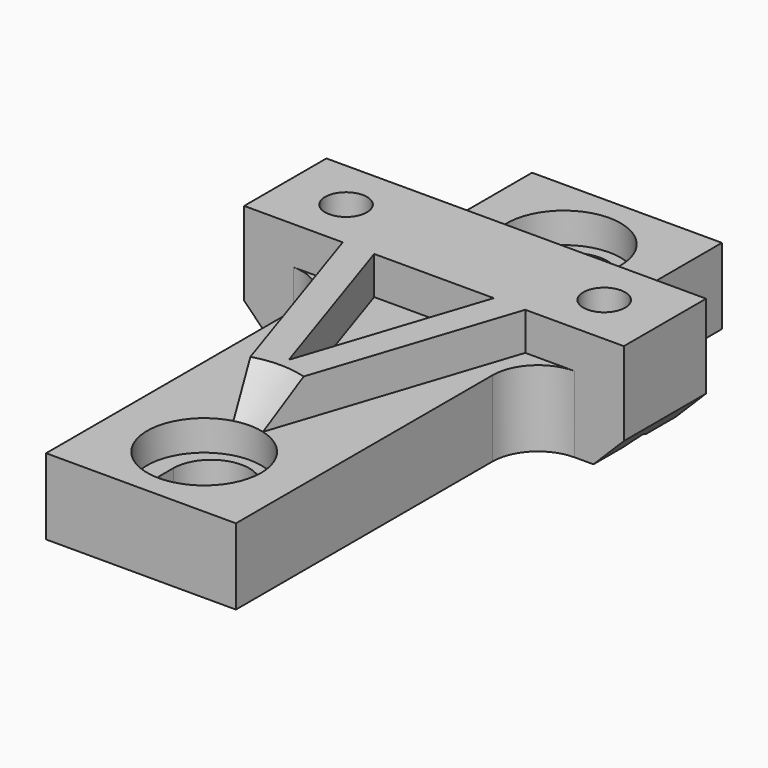
from build123d import *

# Parameters (mm, degrees)
F0_W          = 15.875
F0_H          = 50.8
F1_DEPTH      = 6.35
F2_W          = 31.75
F2_H          = 8.6
F2_R          = 1.75
F3_DEPTH      = 3.175
F3_DEPTH_BACK = 6.35
F4_R          = 4.7625
F5_DEPTH      = 2.54
F6_SIZE       = 2.54
F8_DEPTH      = 5.08
F9_R          = 3.81
F11_DEPTH     = 3.175
F12_SIZE      = 3.17499


# Not quite as in the source:
# - a fillet or chamfer is up to 0.001 mm smaller than in the source, because OpenCascade refuses the exact size


with BuildPart() as f1:
    # F0 (on Top) → F1 (new body)
    with BuildSketch(Plane.XY):
        Rectangle(F0_W, F0_H)
        with BuildLine():
            ThreePointArc((-3.175, -18.058110271), (0.0514516208, -14.8835271912), (3.1733324288, -18.161))
            Line((3.1733324288, -18.161), (3.1733324288, -19.431))
            ThreePointArc((3.1733324288, -19.431), (-0.053119192, -22.6055830798), (-3.175, -19.328110271))
            Line((-3.175, -19.328110271), (-3.175, -18.058110271))
        make_face(mode=Mode.SUBTRACT)
        with BuildLine():
            ThreePointArc((3.1733324288, 18.161), (0.0514516208, 14.8835271912), (-3.175, 18.058110271))
            Line((-3.175, 18.058110271), (-3.175, 19.328110271))
            ThreePointArc((-3.175, 19.328110271), (-0.053119192, 22.6055830798), (3.1733324288, 19.431))
            Line((3.1733324288, 19.431), (3.1733324288, 18.161))
        make_face(mode=Mode.SUBTRACT)
    extrude(amount=F1_DEPTH)

    # F2 (on face) → F3 (join, two sides)
    with BuildSketch(Plane.XY.offset(6.35)) as f3_sk:
        with Locations((0, 9.525)):
            Rectangle(F2_W, F2_H)
        with Locations((-10.795, 9.525)):
            Circle(F2_R, mode=Mode.SUBTRACT)
        with Locations((10.795, 9.525)):
            Circle(F2_R, mode=Mode.SUBTRACT)
    extrude(amount=F3_DEPTH)
    extrude(f3_sk.sketch, amount=-F3_DEPTH_BACK)

    # F4 (on face) → F5 (cut)
    with BuildSketch(Plane.XY.offset(6.35)):
        with Locations((0, -18.796)):
            Circle(F4_R)
        with Locations((0, 18.796)):
            Circle(F4_R)
    extrude(amount=-F5_DEPTH, mode=Mode.SUBTRACT)

    # F6
    f6_edges = [f1.edges().sort_by_distance(p)[0] for p in [
        (-15.875, 9.525, 0),
        (15.875, 9.525, 0),
    ]]
    chamfer(f6_edges, length=F6_SIZE)

    # F7 (on face) → F8 (cut)
    with BuildSketch(Plane(origin=(0, 0, 0), x_dir=(1, 0, 0), z_dir=(0, 0, -1))):
        Polygon((-9.1818833479, -12.319), (-7.5687666958, -9.525), (-9.1818833479, -6.731), (-12.4081166521, -6.731), (-14.0212333042, -9.525), (-12.4081166521, -12.319), align=None)
        Polygon((12.4081166521, -6.731), (9.1818833479, -6.731), (7.5687666958, -9.525), (9.1818833479, -12.319), (12.4081166521, -12.319), (14.0212333042, -9.525), align=None)
    extrude(amount=-F8_DEPTH, mode=Mode.SUBTRACT)

    # F9
    f9_edges = [f1.edges().sort_by_distance(p)[0] for p in [
        (-7.9375, 5.225, 3.175),
        (7.9375, 5.225, 3.175),
        (7.9375, 13.825, 3.175),
        (-7.9375, 13.825, 3.175),
    ]]
    fillet(f9_edges, radius=F9_R)

    # F10 (on face) → F11 (join, through all)
    with BuildSketch(Plane.XY.offset(6.35)):
        with BuildLine():
            Line((-5, 5.225), (-7.6321601122, 5.225))
            Line((-7.6321601122, 5.225), (-1.2342699774, -14.1962191495))
            ThreePointArc((-1.2342699774, -14.1962191495), (0, -14.0335), (1.2342699774, -14.1962191495))
            Line((1.2342699774, -14.1962191495), (7.6321601122, 5.225))
            Line((7.6321601122, 5.225), (5, 5.225))
            Line((5, 5.225), (0, -9.952831082))
            Line((0, -9.952831082), (-5, 5.225))
        make_face()
    extrude(amount=F11_DEPTH)

    # F12 (size 3.175 in the source; OpenCascade refuses exactly that, so slightly less here)
    f12_edges = [f1.edges().sort_by_distance(p)[0] for p in [
        (0, -14.0335, 9.525),
    ]]
    chamfer(f12_edges, length=F12_SIZE)


solid = f1.part
